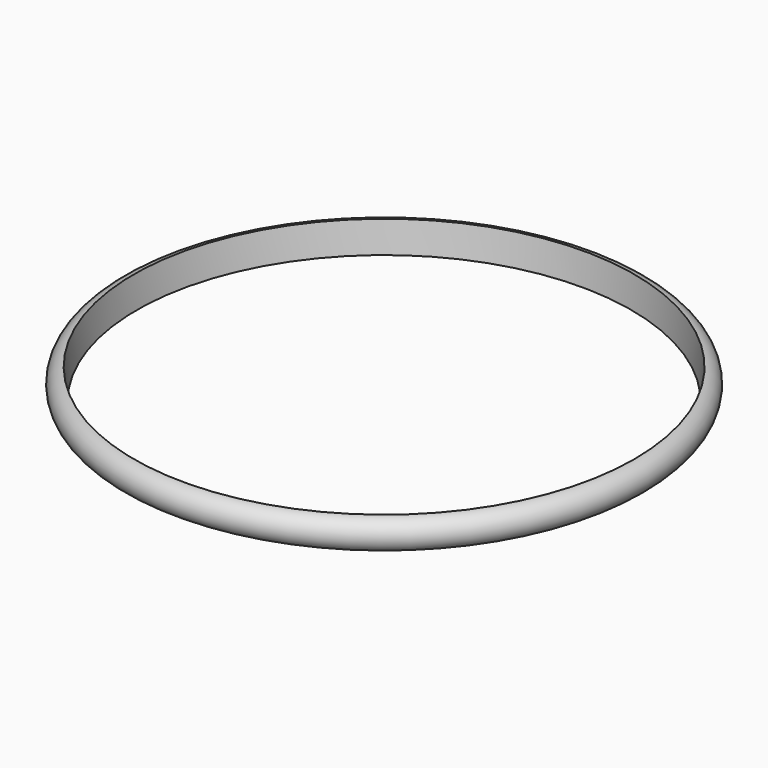
from build123d import *


# Not quite as in the source:
# - the program builds the solid bodies; features that only make, move or delete a surface that nothing else refers to are left out


with BuildPart() as f3:
    # F0 (on Front) → F3 (revolve)
    with BuildSketch(Plane.XZ):
        with BuildLine():
            Line((40.9999983762, 46.5332240357), (40.4949479532, 41.5587970265))
            ThreePointArc((40.4949479532, 41.5587970265), (43.2346866693, 43.7934853196), (40.9999983762, 46.5332240357))
        make_face()
    revolve(axis=Axis((0, 0, 5.4605058394), (0, 0, -1)))


solid = f3.part
